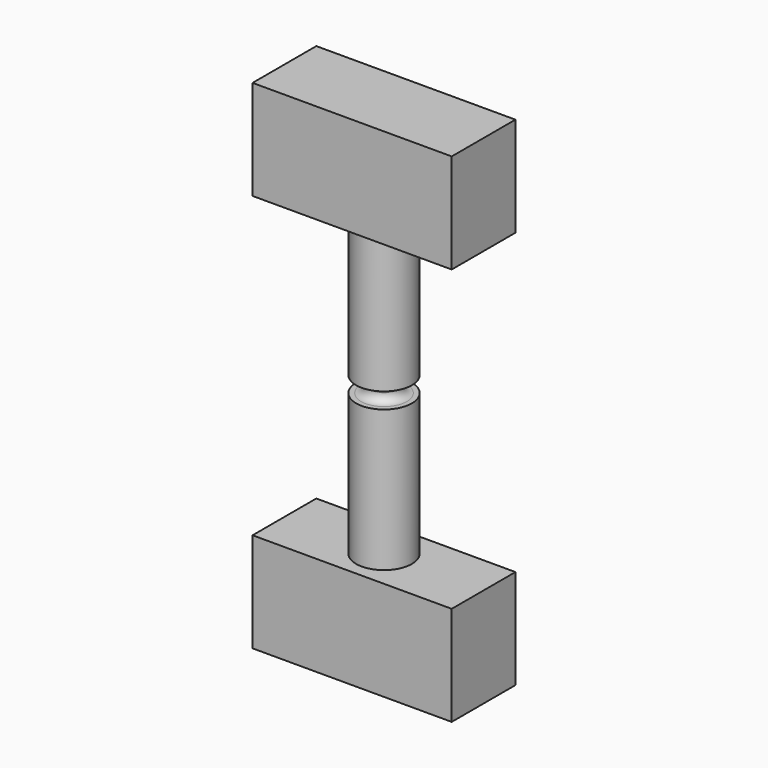
from build123d import *

# Parameters (mm, degrees)
F2_W     = 10
F2_H     = 4
F2_R     = 1.4
F3_DEPTH = 5
F4_W     = 10
F4_H     = 4
F4_R     = 1.4
F5_DEPTH = 5


with BuildPart() as f1:
    # F0 (on Front) → F1 (revolve)
    with BuildSketch(Plane.XZ):
        with BuildLine():
            Line((1.4, 7.5), (0, 7.5))
            Line((0, 7.5), (0, 0))
            Line((0, 0), (0, -7.5))
            Line((0, -7.5), (1.4, -7.5))
            Line((1.4, -7.5), (1.4, -0.4))
            Line((1.4, -0.4), (1.15, -0.4))
            ThreePointArc((1.15, -0.4), (0.8671572875, -0.2828427125), (0.75, 0))
            ThreePointArc((0.75, 0), (0.8671572875, 0.2828427125), (1.15, 0.4))
            Line((1.15, 0.4), (1.4, 0.4))
            Line((1.4, 0.4), (1.4, 7.5))
        make_face()
    revolve(axis=Axis((0, 0, 3.75), (0, 0, 1)))

    # F2 (on face) → F3 (join)
    with BuildSketch(Plane.XY.offset(7.5)):
        Rectangle(F2_W, F2_H)
        Circle(F2_R, mode=Mode.SUBTRACT)
        Circle(F2_R)
    extrude(amount=F3_DEPTH)

    # F4 (on face) → F5 (join)
    with BuildSketch(Plane(origin=(0, 0, -7.5), x_dir=(1, 0, 0), z_dir=(0, 0, -1))):
        Rectangle(F4_W, F4_H)
        Circle(F4_R, mode=Mode.SUBTRACT)
        Circle(F4_R)
    extrude(amount=F5_DEPTH)


solid = f1.part
